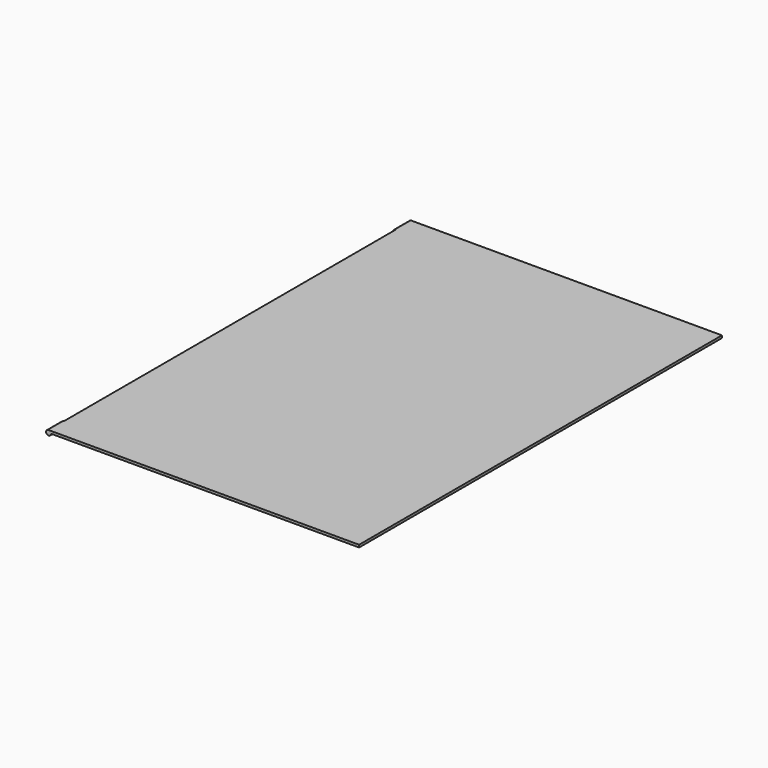
from build123d import *

# Parameters (mm, degrees)
F0_W     = 400.05
F0_H     = 584.2
F1_DEPTH = 3.175
F3_DEPTH = 25.4


with BuildPart() as f1:
    # F0 (on Top) → F1 (new body)
    with BuildSketch(Plane.XY):
        Rectangle(F0_W, F0_H)
    extrude(amount=F1_DEPTH)

    # F2 (on face) → F3 (join)
    with BuildSketch(Plane.XZ.offset(292.1)):
        with BuildLine():
            ThreePointArc((-200.025, 3.175), (-202.2700640303, -2.2450640303), (-196.85, 0))
            Line((-196.85, 0), (-200.025, 0))
            Line((-200.025, 0), (-200.025, 3.175))
        make_face()
    extrude(amount=-F3_DEPTH)

    # F4: F1 across plane


with BuildPart() as f1_1:
    add(f1.part)
    add(f1.part.mirror(Plane.XZ))


solid = f1_1.part
